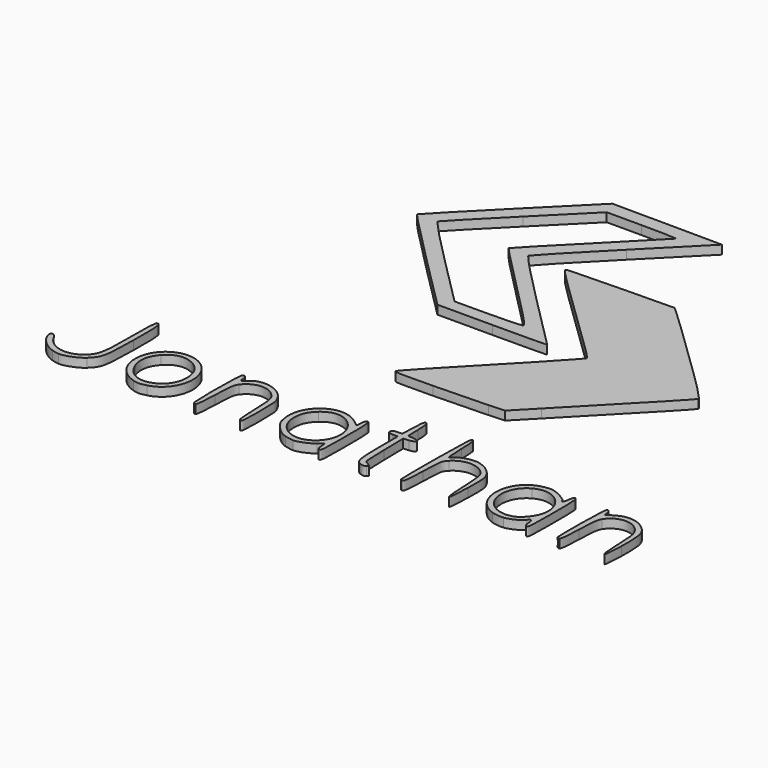
from build123d import *

# Parameters (mm, degrees)
F1_DEPTH = 5


# Not quite as in the source:
# - ends of sketch curves that miss each other by under 0.0002 mm in the source are joined


with BuildPart() as f1:
    # F0 (on Top) → F1 (new body)
    with BuildSketch(Plane.XY):
        with BuildLine():
            add(Edge.make_bspline(
                [(-76.456724, 39.359904), (-93.284564, 56.192016), (-107.052804, 70.323768), (-107.052804, 70.7638)],
                knots=[0, 0, 0, 0, 1, 1, 1, 1], degree=3))
            Line((-76.456724, 39.359904), (-45.860564, 8.756056))
            Line((-45.860564, 8.756056), (-14.723364, 8.756056))
            add(Edge.make_bspline(
                [(16.080556, 9.127536), (16.263836, 8.923224), (2.402076, 8.756056), (-14.723364, 8.756056)],
                knots=[0, 0, 0, 0, 1, 1, 1, 1], degree=3))
            add(Edge.make_bspline(
                [(-14.128964, 39.436632), (2.302956, 22.970944), (15.897196, 9.331848), (16.080556, 9.127536)],
                knots=[0, 0, 0, 0, 1, 1, 1, 1], degree=3))
            add(Edge.make_bspline(
                [(-43.728964, 70.646768), (-43.903684, 69.841728), (-33.029764, 58.37632), (-14.128964, 39.436632)],
                knots=[0, 0, 0, 0, 1, 1, 1, 1], degree=3))
            add(Edge.make_bspline(
                [(-13.452804, 102.137664), (-29.952804, 85.517552), (-43.577044, 71.346648), (-43.728964, 70.646768)],
                knots=[0, 0, 0, 0, 1, 1, 1, 1], degree=3))
            Line((-13.452804, 102.137664), (16.547196, 132.356056))
            Line((16.547196, 132.356056), (-14.639364, 132.565624))
            Line((-14.639364, 132.565624), (-45.826004, 132.775184))
            Line((-45.826004, 132.775184), (-76.439364, 102.16952))
            add(Edge.make_bspline(
                [(-107.052804, 70.7638), (-107.052804, 71.203824), (-93.276804, 85.3364), (-76.439364, 102.16952)],
                knots=[0, 0, 0, 0, 1, 1, 1, 1], degree=3))
        make_face()
        with BuildLine():
            add(Edge.make_bspline(
                [(-3.772564, 16.815728), (-2.929844, 17.344096), (-9.135684, 24.006512), (-28.852804, 43.741416)],
                knots=[0, 0, 0, 0, 1, 1, 1, 1], degree=3))
            add(Edge.make_bspline(
                [(-23.372564, 16.01036), (-13.208404, 16.06716), (-4.388404, 16.429576), (-3.772564, 16.815728)],
                knots=[0, 0, 0, 0, 1, 1, 1, 1], degree=3))
            Line((-23.372564, 16.01036), (-41.852804, 15.907088))
            Line((-41.852804, 15.907088), (-68.951684, 43.034856))
            add(Edge.make_bspline(
                [(-95.740964, 71.091568), (-95.911284, 70.580648), (-83.856084, 57.955128), (-68.951684, 43.034856)],
                knots=[0, 0, 0, 0, 1, 1, 1, 1], degree=3))
            add(Edge.make_bspline(
                [(-69.056964, 98.38828), (-83.562884, 83.886), (-95.570644, 71.60248), (-95.740964, 71.091568)],
                knots=[0, 0, 0, 0, 1, 1, 1, 1], degree=3))
            Line((-69.056964, 98.38828), (-42.682564, 124.756056))
            Line((-42.682564, 124.756056), (-22.867684, 124.756056))
            add(Edge.make_bspline(
                [(-3.052804, 124.15144), (-3.052804, 124.483976), (-11.969524, 124.756056), (-22.867684, 124.756056)],
                knots=[0, 0, 0, 0, 1, 1, 1, 1], degree=3))
            add(Edge.make_bspline(
                [(-29.052804, 97.556056), (-14.752804, 111.850976), (-3.052804, 123.818896), (-3.052804, 124.15144)],
                knots=[0, 0, 0, 0, 1, 1, 1, 1], degree=3))
            add(Edge.make_bspline(
                [(-55.052804, 70.765152), (-55.052804, 71.205224), (-43.352804, 83.261128), (-29.052804, 97.556056)],
                knots=[0, 0, 0, 0, 1, 1, 1, 1], degree=3))
            add(Edge.make_bspline(
                [(-28.852804, 43.741416), (-43.262804, 58.164392), (-55.052804, 70.325072), (-55.052804, 70.765152)],
                knots=[0, 0, 0, 0, 1, 1, 1, 1], degree=3))
        make_face(mode=Mode.SUBTRACT)
    extrude(amount=F1_DEPTH)


with BuildPart() as f1b:
    # F0 (on Top) → F1, piece 2 (new body)
    with BuildSketch(Plane.XY):
        with BuildLine():
            add(Edge.make_bspline(
                [(-20.508244, -52.49384), (-20.269684, -51.450352), (-11.723684, -42.3928), (23.547196, -5.80124)],
                knots=[0, 0, 0, 0, 1, 1, 1, 1], degree=3))
            add(Edge.make_bspline(
                [(1.091756, -53.202624), (-17.353764, -53.54736), (-20.723924, -53.436768), (-20.508244, -52.49384)],
                knots=[0, 0, 0, 0, 1, 1, 1, 1], degree=3))
            add(Edge.make_bspline(
                [(31.931276, -52.341264), (26.989996, -52.59036), (13.112236, -52.977976), (1.091756, -53.202624)],
                knots=[0, 0, 0, 0, 1, 1, 1, 1], degree=3))
            Line((31.931276, -52.341264), (40.915356, -51.888352))
            Line((40.915356, -51.888352), (52.331276, -40.16672))
            add(Edge.make_bspline(
                [(100.772156, 10.620664), (100.502076, 9.438136), (93.851116, 2.465008), (52.331276, -40.16672)],
                knots=[0, 0, 0, 0, 1, 1, 1, 1], degree=3))
            add(Edge.make_bspline(
                [(82.788156, 29.180744), (92.803116, 19.514464), (100.895836, 11.162432), (100.772156, 10.620664)],
                knots=[0, 0, 0, 0, 1, 1, 1, 1], degree=3))
            add(Edge.make_bspline(
                [(53.763196, 57.263816), (59.712076, 51.484408), (72.773276, 38.847024), (82.788156, 29.180744)],
                knots=[0, 0, 0, 0, 1, 1, 1, 1], degree=3))
            add(Edge.make_bspline(
                [(40.437116, 69.859296), (41.817676, 68.711184), (47.814396, 63.043216), (53.763196, 57.263816)],
                knots=[0, 0, 0, 0, 1, 1, 1, 1], degree=3))
            Line((40.437116, 69.859296), (37.926956, 71.94676))
            Line((37.926956, 71.94676), (9.637116, 71.508768))
            add(Edge.make_bspline(
                [(-21.140324, 70.698144), (-19.772164, 70.903096), (-5.922324, 71.26788), (9.637116, 71.508768)],
                knots=[0, 0, 0, 0, 1, 1, 1, 1], degree=3))
            add(Edge.make_bspline(
                [(-11.543284, 58.540656), (-23.509924, 70.210584), (-23.603524, 70.329144), (-21.140324, 70.698144)],
                knots=[0, 0, 0, 0, 1, 1, 1, 1], degree=3))
            add(Edge.make_bspline(
                [(30.747196, 17.536656), (24.015756, 23.917336), (14.429596, 33.211912), (-11.543284, 58.540656)],
                knots=[0, 0, 0, 0, 1, 1, 1, 1], degree=3))
            add(Edge.make_bspline(
                [(37.747196, 9.915936), (37.747196, 10.457944), (34.597196, 13.887272), (30.747196, 17.536656)],
                knots=[0, 0, 0, 0, 1, 1, 1, 1], degree=3))
            add(Edge.make_bspline(
                [(23.547196, -5.80124), (31.357196, 2.301192), (37.747196, 9.373928), (37.747196, 9.915936)],
                knots=[0, 0, 0, 0, 1, 1, 1, 1], degree=3))
        make_face()
    extrude(amount=F1_DEPTH)


with BuildPart() as f1c:
    # F0 (on Top) → F1, piece 3 (new body)
    with BuildSketch(Plane.XY):
        with BuildLine():
            add(Edge.make_bspline(
                [(-151.334004, -132.022648), (-156.287844, -130.537784), (-161.730404, -125.246728), (-162.391444, -121.272944)],
                knots=[0, 0, 0, 0, 1, 1, 1, 1], degree=3))
            add(Edge.make_bspline(
                [(-147.398004, -132.775184), (-148.308164, -132.737344), (-150.079364, -132.39872), (-151.334004, -132.022648)],
                knots=[0, 0, 0, 0, 1, 1, 1, 1], degree=3))
            add(Edge.make_bspline(
                [(-135.107204, -127.864208), (-137.723204, -130.411608), (-143.992724, -132.91668), (-147.398004, -132.775184)],
                knots=[0, 0, 0, 0, 1, 1, 1, 1], degree=3))
            add(Edge.make_bspline(
                [(-129.655604, -102.043944), (-129.948084, -121.507208), (-130.302484, -123.185448), (-135.107204, -127.864208)],
                knots=[0, 0, 0, 0, 1, 1, 1, 1], degree=3))
            add(Edge.make_bspline(
                [(-131.763364, -82.788664), (-129.786084, -81.566624), (-129.400724, -85.08688), (-129.655604, -102.043944)],
                knots=[0, 0, 0, 0, 1, 1, 1, 1], degree=3))
            add(Edge.make_bspline(
                [(-132.657284, -99.89116), (-132.657284, -88.613688), (-132.369364, -83.163184), (-131.763364, -82.788664)],
                knots=[0, 0, 0, 0, 1, 1, 1, 1], degree=3))
            add(Edge.make_bspline(
                [(-136.975204, -125.326336), (-133.208404, -121.559504), (-132.662244, -118.342488), (-132.657284, -99.89116)],
                knots=[0, 0, 0, 0, 1, 1, 1, 1], degree=3))
            add(Edge.make_bspline(
                [(-158.652804, -122.20504), (-154.323204, -130.294256), (-143.501284, -131.852464), (-136.975204, -125.326336)],
                knots=[0, 0, 0, 0, 1, 1, 1, 1], degree=3))
            add(Edge.make_bspline(
                [(-162.391444, -121.272944), (-162.863444, -118.43592), (-160.332404, -119.066928), (-158.652804, -122.20504)],
                knots=[0, 0, 0, 0, 1, 1, 1, 1], degree=3))
        make_face()
    extrude(amount=F1_DEPTH)


with BuildPart() as f1d:
    # F0 (on Top) → F1, piece 4 (new body)
    with BuildSketch(Plane.XY):
        with BuildLine():
            add(Edge.make_bspline(
                [(-105.641604, -132.047368), (-105.6417025353, -132.0473383304), (-105.6418010703, -132.0473086598), (-105.6418996051, -132.0472789882)],
                knots=[0, 0, 0, 0, 2.38335e-05, 2.38335e-05, 2.38335e-05, 2.38335e-05], degree=3))
            add(Edge.make_bspline(
                [(-97.903924, -131.97328), (-101.825397617, -132.9607201763), (-102.5842750884, -132.9680155308), (-105.641604, -132.047368)],
                knots=[0, 0, 0, 0, 0.9999677726, 0.9999677726, 0.9999677726, 0.9999677726], degree=3))
            add(Edge.make_bspline(
                [(-91.621524, -101.713624), (-81.010564, -110.460072), (-84.791604, -128.671544), (-97.903924, -131.97328)],
                knots=[0, 0, 0, 0, 1, 1, 1, 1], degree=3))
            add(Edge.make_bspline(
                [(-115.631844, -106.2652), (-110.529844, -97.585848), (-99.228324, -95.443448), (-91.621524, -101.713624)],
                knots=[0, 0, 0, 0, 1, 1, 1, 1], degree=3))
            add(Edge.make_bspline(
                [(-115.659844, -124.174312), (-118.789924, -118.849736), (-118.778484, -111.618736), (-115.631844, -106.2652)],
                knots=[0, 0, 0, 0, 1, 1, 1, 1], degree=3))
            add(Edge.make_bspline(
                [(-105.6418996051, -132.0472789882), (-109.7761000886, -130.8023576162), (-113.4701361896, -127.8992792189), (-115.659844, -124.174312)],
                knots=[2.38335e-05, 2.38335e-05, 2.38335e-05, 2.38335e-05, 1, 1, 1, 1], degree=3))
        make_face()
        with BuildLine():
            add(Edge.make_bspline(
                [(-96.094084, -127.967096), (-86.108484, -123.133144), (-86.108484, -107.354728), (-96.094084, -102.520776)],
                knots=[0, 0, 0, 0, 1, 1, 1, 1], degree=3))
            add(Edge.make_bspline(
                [(-113.814644, -120.658712), (-110.479524, -128.640728), (-103.463204, -131.534432), (-96.094084, -127.967096)],
                knots=[0, 0, 0, 0, 1, 1, 1, 1], degree=3))
            add(Edge.make_bspline(
                [(-111.201924, -105.345408), (-115.167924, -109.587176), (-116.116804, -115.148752), (-113.814644, -120.658712)],
                knots=[0, 0, 0, 0, 1, 1, 1, 1], degree=3))
            add(Edge.make_bspline(
                [(-96.094084, -102.520776), (-101.772084, -99.77212), (-106.884644, -100.728), (-111.201924, -105.345408)],
                knots=[0, 0, 0, 0, 1, 1, 1, 1], degree=3))
        make_face(mode=Mode.SUBTRACT)
    extrude(amount=F1_DEPTH)


with BuildPart() as f1e:
    # F0 (on Top) → F1, piece 5 (new body)
    with BuildSketch(Plane.XY):
        with BuildLine():
            add(Edge.make_bspline(
                [(-71.354244, -131.61232), (-72.122404, -129.610464), (-71.920244, -99.78904), (-71.130004, -98.54144)],
                knots=[0, 0, 0, 0, 1, 1, 1, 1], degree=3))
            add(Edge.make_bspline(
                [(-69.954244, -132.613352), (-70.450004, -132.777368), (-71.080004, -132.326904), (-71.354244, -131.61232)],
                knots=[0, 0, 0, 0, 1, 1, 1, 1], degree=3))
            add(Edge.make_bspline(
                [(-68.652804, -120.235032), (-68.915204, -128.158584), (-69.362964, -132.417752), (-69.954244, -132.613352)],
                knots=[0, 0, 0, 0, 1, 1, 1, 1], degree=3))
            add(Edge.make_bspline(
                [(-66.595924, -105.899432), (-68.047204, -107.875048), (-68.302404, -109.653912), (-68.652804, -120.235032)],
                knots=[0, 0, 0, 0, 1, 1, 1, 1], degree=3))
            add(Edge.make_bspline(
                [(-48.063924, -106.215984), (-52.447284, -99.53836), (-61.805684, -99.378504), (-66.595924, -105.899432)],
                knots=[0, 0, 0, 0, 1, 1, 1, 1], degree=3))
            add(Edge.make_bspline(
                [(-46.252804, -120.40484), (-46.574484, -110.722216), (-46.929044, -107.94496), (-48.063924, -106.215984)],
                knots=[0, 0, 0, 0, 1, 1, 1, 1], degree=3))
            add(Edge.make_bspline(
                [(-44.652804, -132.443936), (-45.648564, -132.443936), (-45.920884, -130.395144), (-46.252804, -120.40484)],
                knots=[0, 0, 0, 0, 1, 1, 1, 1], degree=3))
            add(Edge.make_bspline(
                [(-43.452804, -120.443936), (-43.452804, -130.577272), (-43.639444, -132.443936), (-44.652804, -132.443936)],
                knots=[0, 0, 0, 0, 1, 1, 1, 1], degree=3))
            add(Edge.make_bspline(
                [(-45.347124, -105.138248), (-43.585844, -108.211824), (-43.452804, -109.286512), (-43.452804, -120.443936)],
                knots=[0, 0, 0, 0, 1, 1, 1, 1], degree=3))
            add(Edge.make_bspline(
                [(-65.849764, -100.84056), (-61.022084, -95.50604), (-49.480404, -97.92536), (-45.347124, -105.138248)],
                knots=[0, 0, 0, 0, 1, 1, 1, 1], degree=3))
            add(Edge.make_bspline(
                [(-68.652804, -100.491152), (-68.652804, -102.8632), (-67.778804, -102.972144), (-65.849764, -100.84056)],
                knots=[0, 0, 0, 0, 1, 1, 1, 1], degree=3))
            add(Edge.make_bspline(
                [(-71.130004, -98.54144), (-70.146484, -96.98864), (-68.652804, -98.164248), (-68.652804, -100.491152)],
                knots=[0, 0, 0, 0, 1, 1, 1, 1], degree=3))
        make_face()
    extrude(amount=F1_DEPTH)


with BuildPart() as f1f:
    # F0 (on Top) → F1, piece 6 (new body)
    with BuildSketch(Plane.XY):
        with BuildLine():
            add(Edge.make_bspline(
                [(-19.384484, -131.850648), (-23.438324, -130.778904), (-29.056404, -125.20152), (-30.188404, -121.124968)],
                knots=[0, 0, 0, 0, 1, 1, 1, 1], degree=3))
            add(Edge.make_bspline(
                [(-14.652804, -132.726136), (-15.532804, -132.699976), (-17.662084, -132.306008), (-19.384484, -131.850648)],
                knots=[0, 0, 0, 0, 1, 1, 1, 1], degree=3))
            add(Edge.make_bspline(
                [(-4.299684, -128.533936), (-7.324964, -130.84144), (-12.162324, -132.800184), (-14.652804, -132.726136)],
                knots=[0, 0, 0, 0, 1, 1, 1, 1], degree=3))
            Line((-4.299684, -128.533936), (-1.549844, -126.436512))
            Line((-1.549844, -126.436512), (-1.301284, -129.440224))
            add(Edge.make_bspline(
                [(0.147196, -132.443936), (-0.662244, -132.443936), (-1.133684, -131.466408), (-1.301284, -129.440224)],
                knots=[0, 0, 0, 0, 1, 1, 1, 1], degree=3))
            add(Edge.make_bspline(
                [(1.347196, -115.243936), (1.347196, -129.999488), (1.176636, -132.443936), (0.147196, -132.443936)],
                knots=[0, 0, 0, 0, 1, 1, 1, 1], degree=3))
            add(Edge.make_bspline(
                [(0.147196, -98.043936), (1.176636, -98.043936), (1.347196, -100.488384), (1.347196, -115.243936)],
                knots=[0, 0, 0, 0, 1, 1, 1, 1], degree=3))
            add(Edge.make_bspline(
                [(-1.301044, -101.04288), (-1.133684, -99.020808), (-0.661924, -98.043936), (0.147196, -98.043936)],
                knots=[0, 0, 0, 0, 1, 1, 1, 1], degree=3))
            Line((-1.301044, -101.04288), (-1.549284, -104.041816))
            Line((-1.549284, -104.041816), (-4.501044, -101.704736))
            add(Edge.make_bspline(
                [(-25.801604, -102.75556), (-19.845604, -96.79064), (-11.243604, -96.36628), (-4.501044, -101.704736)],
                knots=[0, 0, 0, 0, 1, 1, 1, 1], degree=3))
            add(Edge.make_bspline(
                [(-30.188404, -121.124968), (-32.156644, -114.036424), (-30.613524, -107.574712), (-25.801604, -102.75556)],
                knots=[0, 0, 0, 0, 1, 1, 1, 1], degree=3))
        make_face()
        with BuildLine():
            add(Edge.make_bspline(
                [(-10.027124, -128.542464), (-0.304004, -124.382224), (1.577036, -111.377144), (-6.516564, -104.270896)],
                knots=[0, 0, 0, 0, 1, 1, 1, 1], degree=3))
            add(Edge.make_bspline(
                [(-27.852804, -115.657928), (-27.852804, -125.234904), (-18.350004, -132.10356), (-10.027124, -128.542464)],
                knots=[0, 0, 0, 0, 1, 1, 1, 1], degree=3))
            add(Edge.make_bspline(
                [(-22.831364, -104.308016), (-26.327044, -107.377256), (-27.852804, -110.825888), (-27.852804, -115.657928)],
                knots=[0, 0, 0, 0, 1, 1, 1, 1], degree=3))
            add(Edge.make_bspline(
                [(-6.516564, -104.270896), (-11.575844, -99.828736), (-17.745764, -99.842784), (-22.831364, -104.308016)],
                knots=[0, 0, 0, 0, 1, 1, 1, 1], degree=3))
        make_face(mode=Mode.SUBTRACT)
    extrude(amount=F1_DEPTH)


with BuildPart() as f1g:
    # F0 (on Top) → F1, piece 7 (new body)
    with BuildSketch(Plane.XY):
        with BuildLine():
            add(Edge.make_bspline(
                [(23.262796, -131.908384), (19.884556, -130.740312), (19.347196, -128.283448), (19.347196, -114.006304)],
                knots=[0, 0, 0, 0, 1, 1, 1, 1], degree=3))
            add(Edge.make_bspline(
                [(26.366636, -131.822528), (25.725276, -132.330024), (24.574396, -132.361864), (23.262796, -131.908384)],
                knots=[0, 0, 0, 0, 1, 1, 1, 1], degree=3))
            add(Edge.make_bspline(
                [(24.761436, -129.302008), (27.311356, -130.572064), (27.524316, -130.906464), (26.366636, -131.822528)],
                knots=[0, 0, 0, 0, 1, 1, 1, 1], degree=3))
            add(Edge.make_bspline(
                [(22.728636, -114.670576), (22.941516, -128.03616), (22.995116, -128.422248), (24.761436, -129.302008)],
                knots=[0, 0, 0, 0, 1, 1, 1, 1], degree=3))
            Line((22.728636, -114.670576), (22.509916, -100.942752))
            Line((22.509916, -100.942752), (25.528636, -100.693352))
            add(Edge.make_bspline(
                [(25.576636, -97.797408), (29.701196, -98.13972), (29.664476, -100.351632), (25.528636, -100.693352)],
                knots=[0, 0, 0, 0, 1, 1, 1, 1], degree=3))
            Line((25.576636, -97.797408), (22.605996, -97.550864))
            Line((22.605996, -97.550864), (22.376636, -90.197408))
            add(Edge.make_bspline(
                [(20.947196, -82.843944), (21.910156, -82.843944), (22.192476, -84.296288), (22.376636, -90.197408)],
                knots=[0, 0, 0, 0, 1, 1, 1, 1], degree=3))
            add(Edge.make_bspline(
                [(19.517196, -90.243944), (19.701916, -84.301728), (19.983596, -82.843944), (20.947196, -82.843944)],
                knots=[0, 0, 0, 0, 1, 1, 1, 1], degree=3))
            Line((19.517196, -90.243944), (19.287116, -97.643944))
            Line((19.287116, -97.643944), (16.517196, -97.643944))
            add(Edge.make_bspline(
                [(13.747196, -99.243944), (13.747196, -97.952008), (14.280556, -97.643944), (16.517196, -97.643944)],
                knots=[0, 0, 0, 0, 1, 1, 1, 1], degree=3))
            add(Edge.make_bspline(
                [(16.547196, -100.843944), (14.280556, -100.843944), (13.747196, -100.539184), (13.747196, -99.243944)],
                knots=[0, 0, 0, 0, 1, 1, 1, 1], degree=3))
            Line((16.547196, -100.843944), (19.347196, -100.843944))
            Line((19.347196, -100.843944), (19.347196, -114.006304))
        make_face()
    extrude(amount=F1_DEPTH)


with BuildPart() as f1h:
    # F0 (on Top) → F1, piece 8 (new body)
    with BuildSketch(Plane.XY):
        with BuildLine():
            add(Edge.make_bspline(
                [(46.135436, -131.901984), (45.908476, -131.310584), (45.818316, -120.030648), (45.935036, -106.835456)],
                knots=[0, 0, 0, 0, 1, 1, 1, 1], degree=3))
            add(Edge.make_bspline(
                [(47.547596, -132.646248), (46.997836, -132.828304), (46.362396, -132.493384), (46.135436, -131.901984)],
                knots=[0, 0, 0, 0, 1, 1, 1, 1], degree=3))
            add(Edge.make_bspline(
                [(48.947196, -119.82988), (48.659436, -128.810672), (48.266636, -132.40816), (47.547596, -132.646248)],
                knots=[0, 0, 0, 0, 1, 1, 1, 1], degree=3))
            add(Edge.make_bspline(
                [(51.679116, -104.912848), (49.349836, -107.341752), (49.346716, -107.358664), (48.947196, -119.82988)],
                knots=[0, 0, 0, 0, 1, 1, 1, 1], degree=3))
            add(Edge.make_bspline(
                [(70.715276, -106.70624), (67.061516, -100.077648), (57.206476, -99.1492), (51.679116, -104.912848)],
                knots=[0, 0, 0, 0, 1, 1, 1, 1], degree=3))
            add(Edge.make_bspline(
                [(72.110236, -120.252144), (71.857596, -113.424648), (71.269196, -107.711152), (70.715276, -106.70624)],
                knots=[0, 0, 0, 0, 1, 1, 1, 1], degree=3))
            add(Edge.make_bspline(
                [(74.368316, -119.992632), (74.077596, -135.842512), (72.693036, -136.001632), (72.110236, -120.252144)],
                knots=[0, 0, 0, 0, 1, 1, 1, 1], degree=3))
            add(Edge.make_bspline(
                [(72.873996, -104.885016), (74.449996, -107.689104), (74.571436, -108.917208), (74.368316, -119.992632)],
                knots=[0, 0, 0, 0, 1, 1, 1, 1], degree=3))
            add(Edge.make_bspline(
                [(62.881196, -98.09704), (67.088476, -98.986104), (71.084076, -101.70028), (72.873996, -104.885016)],
                knots=[0, 0, 0, 0, 1, 1, 1, 1], degree=3))
            add(Edge.make_bspline(
                [(51.819516, -100.776264), (53.989276, -98.737872), (59.545436, -97.392136), (62.881196, -98.09704)],
                knots=[0, 0, 0, 0, 1, 1, 1, 1], degree=3))
            add(Edge.make_bspline(
                [(49.520236, -102.4442), (49.808396, -102.4442), (50.843036, -101.693632), (51.819516, -100.776264)],
                knots=[0, 0, 0, 0, 1, 1, 1, 1], degree=3))
            add(Edge.make_bspline(
                [(48.771836, -92.6442), (48.895356, -98.0342), (49.232156, -102.4442), (49.520236, -102.4442)],
                knots=[0, 0, 0, 0, 1, 1, 1, 1], degree=3))
            add(Edge.make_bspline(
                [(47.347196, -82.8442), (48.336316, -82.8442), (48.586636, -84.566256), (48.771836, -92.6442)],
                knots=[0, 0, 0, 0, 1, 1, 1, 1], degree=3))
            add(Edge.make_bspline(
                [(45.935036, -106.835456), (46.118076, -86.137536), (46.311916, -82.8442), (47.347196, -82.8442)],
                knots=[0, 0, 0, 0, 1, 1, 1, 1], degree=3))
        make_face()
    extrude(amount=F1_DEPTH)


with BuildPart() as f1i:
    # F0 (on Top) → F1, piece 9 (new body)
    with BuildSketch(Plane.XY):
        with BuildLine():
            add(Edge.make_bspline(
                [(97.848716, -131.681456), (82.506636, -126.740864), (82.863356, -103.252904), (98.348876, -98.75116)],
                knots=[0, 0, 0, 0, 1, 1, 1, 1], degree=3))
            add(Edge.make_bspline(
                [(104.547196, -132.38576), (102.766236, -132.620792), (99.795756, -132.30848), (97.848716, -131.681456)],
                knots=[0, 0, 0, 0, 1, 1, 1, 1], degree=3))
            add(Edge.make_bspline(
                [(113.986956, -127.561496), (112.936636, -129.395848), (107.970076, -131.934032), (104.547196, -132.38576)],
                knots=[0, 0, 0, 0, 1, 1, 1, 1], degree=3))
            add(Edge.make_bspline(
                [(116.298876, -129.4442), (116.043356, -126.356576), (115.111436, -125.597664), (113.986956, -127.561496)],
                knots=[0, 0, 0, 0, 1, 1, 1, 1], degree=3))
            add(Edge.make_bspline(
                [(117.747196, -132.4442), (116.937996, -132.4442), (116.466316, -131.467184), (116.298876, -129.4442)],
                knots=[0, 0, 0, 0, 1, 1, 1, 1], degree=3))
            add(Edge.make_bspline(
                [(118.947196, -115.2442), (118.947196, -129.999752), (118.776636, -132.4442), (117.747196, -132.4442)],
                knots=[0, 0, 0, 0, 1, 1, 1, 1], degree=3))
            add(Edge.make_bspline(
                [(117.747196, -98.0442), (118.776636, -98.0442), (118.947196, -100.488648), (118.947196, -115.2442)],
                knots=[0, 0, 0, 0, 1, 1, 1, 1], degree=3))
            add(Edge.make_bspline(
                [(116.298876, -101.0442), (116.466316, -99.021216), (116.937996, -98.0442), (117.747196, -98.0442)],
                knots=[0, 0, 0, 0, 1, 1, 1, 1], degree=3))
            add(Edge.make_bspline(
                [(115.298876, -104.0442), (115.712316, -104.0442), (116.162316, -102.6942), (116.298876, -101.0442)],
                knots=[0, 0, 0, 0, 1, 1, 1, 1], degree=3))
            add(Edge.make_bspline(
                [(114.547196, -103.27792), (114.547196, -103.699376), (114.885436, -104.0442), (115.298876, -104.0442)],
                knots=[0, 0, 0, 0, 1, 1, 1, 1], degree=3))
            add(Edge.make_bspline(
                [(105.160476, -98.061992), (108.262396, -98.70844), (114.547196, -102.200728), (114.547196, -103.27792)],
                knots=[0, 0, 0, 0, 1, 1, 1, 1], degree=3))
            add(Edge.make_bspline(
                [(98.348876, -98.75116), (100.883516, -98.014304), (103.608716, -97.738592), (105.160476, -98.061992)],
                knots=[0, 0, 0, 0, 1, 1, 1, 1], degree=3))
        make_face()
        with BuildLine():
            add(Edge.make_bspline(
                [(109.638556, -127.458608), (110.798316, -126.599768), (112.548396, -124.719952), (113.527756, -123.28124)],
                knots=[0, 0, 0, 0, 1, 1, 1, 1], degree=3))
            add(Edge.make_bspline(
                [(97.125676, -127.994264), (101.213516, -130.0714), (106.410876, -129.848912), (109.638556, -127.458608)],
                knots=[0, 0, 0, 0, 1, 1, 1, 1], degree=3))
            add(Edge.make_bspline(
                [(96.947196, -102.637552), (87.046716, -107.915072), (87.152396, -122.926584), (97.125676, -127.994264)],
                knots=[0, 0, 0, 0, 1, 1, 1, 1], degree=3))
            add(Edge.make_bspline(
                [(113.527756, -123.28124), (121.542796, -111.505928), (109.181836, -96.115816), (96.947196, -102.637552)],
                knots=[0, 0, 0, 0, 1, 1, 1, 1], degree=3))
        make_face(mode=Mode.SUBTRACT)
    extrude(amount=F1_DEPTH)


with BuildPart() as f1j:
    # F0 (on Top) → F1, piece 10 (new body)
    with BuildSketch(Plane.XY):
        with BuildLine():
            add(Edge.make_bspline(
                [(134.930476, -131.889128), (134.700796, -131.290656), (134.610636, -123.43072), (134.730076, -114.4226)],
                knots=[0, 0, 0, 0, 1, 1, 1, 1], degree=3))
            add(Edge.make_bspline(
                [(136.347596, -132.646072), (135.797836, -132.828224), (135.160156, -132.487592), (134.930476, -131.889128)],
                knots=[0, 0, 0, 0, 1, 1, 1, 1], degree=3))
            add(Edge.make_bspline(
                [(137.747196, -120.339352), (137.460876, -128.911792), (137.063116, -132.409), (136.347596, -132.646072)],
                knots=[0, 0, 0, 0, 1, 1, 1, 1], degree=3))
            add(Edge.make_bspline(
                [(139.558316, -106.215152), (138.424556, -107.941544), (138.068556, -110.717376), (137.747196, -120.339352)],
                knots=[0, 0, 0, 0, 1, 1, 1, 1], degree=3))
            add(Edge.make_bspline(
                [(158.147196, -106.53468), (153.951036, -99.428632), (144.126316, -99.259752), (139.558316, -106.215152)],
                knots=[0, 0, 0, 0, 1, 1, 1, 1], degree=3))
            add(Edge.make_bspline(
                [(160.147196, -120.650592), (159.814156, -111.1532), (159.479436, -108.790728), (158.147196, -106.53468)],
                knots=[0, 0, 0, 0, 1, 1, 1, 1], degree=3))
            add(Edge.make_bspline(
                [(162.391596, -121.046496), (162.064156, -135.788224), (160.669436, -135.5422), (160.147196, -120.650592)],
                knots=[0, 0, 0, 0, 1, 1, 1, 1], degree=3))
            add(Edge.make_bspline(
                [(158.147836, -101.752056), (161.985436, -105.12156), (162.675596, -108.259256), (162.391596, -121.046496)],
                knots=[0, 0, 0, 0, 1, 1, 1, 1], degree=3))
            add(Edge.make_bspline(
                [(140.798156, -100.494968), (146.634236, -96.726064), (152.944236, -97.183264), (158.147836, -101.752056)],
                knots=[0, 0, 0, 0, 1, 1, 1, 1], degree=3))
            Line((140.798156, -100.494968), (137.849116, -102.399432))
            Line((137.849116, -102.399432), (137.598156, -100.221816))
            add(Edge.make_bspline(
                [(136.147196, -98.0442), (136.858476, -98.0442), (137.449436, -98.93104), (137.598156, -100.221816)],
                knots=[0, 0, 0, 0, 1, 1, 1, 1], degree=3))
            add(Edge.make_bspline(
                [(134.730076, -114.4226), (134.914716, -100.493856), (135.126636, -98.0442), (136.147196, -98.0442)],
                knots=[0, 0, 0, 0, 1, 1, 1, 1], degree=3))
        make_face()
    extrude(amount=F1_DEPTH)


solid = Compound([f1.part, f1b.part, f1c.part, f1d.part, f1e.part, f1f.part, f1g.part, f1h.part, f1i.part, f1j.part])
